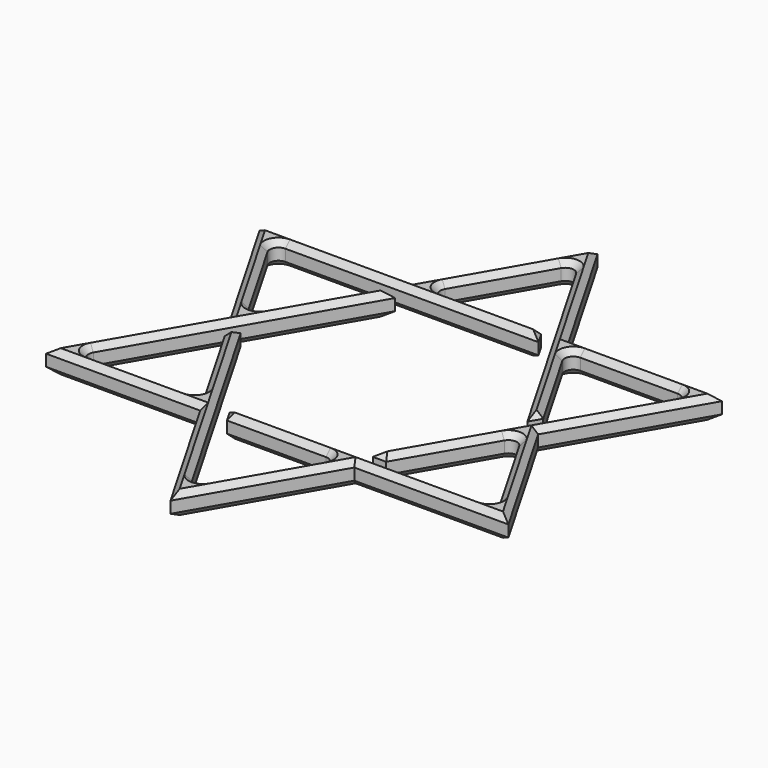
from build123d import *

# Parameters (mm, degrees)
F1_DEPTH = 12.7
F2_SIZE  = 3.17499
F3_SIZE  = 3.17499


# Not quite as in the source:
# - a fillet or chamfer is up to 0.001 mm smaller than in the source, because OpenCascade refuses the exact size


with BuildPart() as f1:
    # F0 (on Top) → F1 (new body)
    with BuildSketch(Plane.XY):
        Polygon((42.3333333333, 73.3234841871), (0, 146.6469683742), (-42.3333333333, 73.3234841871), (-127, 73.3234841871), (-84.6666666667, 0), (-127, -73.3234841871), (-42.3333333333, -73.3234841871), (0, -146.6469683742), (42.3333333333, -73.3234841871), (127, -73.3234841871), (84.6666666667, 0), (127, 73.3234841871), align=None)
        with BuildLine():
            ThreePointArc((107.7525859006, 66.9734850526), (111.8770318861, 64.5922350526), (111.8770318861, 59.8297350526))
            Line((111.8770318861, 59.8297350526), (42.3333325205, -60.623485595))
            Line((42.3333325205, -60.623485595), (49.6656809392, -60.623485595))
            Line((49.6656809392, -60.623485595), (76.8760464718, -13.49375))
            ThreePointArc((76.8760464718, -13.49375), (81.0004924573, -11.1125), (85.1249384428, -13.49375))
            Line((85.1249384428, -13.49375), (111.8770318861, -59.8297350526))
            ThreePointArc((111.8770318861, -59.8297350526), (111.8770318861, -64.5922350526), (107.7525859006, -66.9734850526))
            Line((107.7525859006, -66.9734850526), (-31.3348102056, -66.9734850526))
            Line((-31.3348102056, -66.9734850526), (-27.6686364959, -73.3234841871))
            Line((-27.6686364959, -73.3234841871), (26.7520929436, -73.3234841871))
            ThreePointArc((26.7520929436, -73.3234841871), (30.8765389291, -75.7047341871), (30.8765389291, -80.4672341871))
            Line((30.8765389291, -80.4672341871), (4.1244459855, -126.8032183742))
            ThreePointArc((4.1244459855, -126.8032183742), (0, -129.1844683742), (-4.1244459855, -126.8032183742))
            Line((-4.1244459855, -126.8032183742), (-73.6681446525, -6.3499989368))
            Line((-73.6681446525, -6.3499989368), (-77.3343188618, -12.6999989368))
            Line((-77.3343188618, -12.6999989368), (-50.1239530285, -59.8297350526))
            ThreePointArc((-50.1239530285, -59.8297350526), (-50.1239530285, -64.5922350526), (-54.2483990141, -66.9734850526))
            Line((-54.2483990141, -66.9734850526), (-107.7525871283, -66.9734850526))
            ThreePointArc((-107.7525871283, -66.9734850526), (-111.8770331138, -64.5922350526), (-111.8770331138, -59.8297350526))
            Line((-111.8770331138, -59.8297350526), (-42.3333337482, 60.623485595))
            Line((-42.3333337482, 60.623485595), (-49.6656809392, 60.623485595))
            Line((-49.6656809392, 60.623485595), (-76.8760464718, 13.49375))
            ThreePointArc((-76.8760464718, 13.49375), (-81.0004924573, 11.1125), (-85.1249384428, 13.49375))
            Line((-85.1249384428, 13.49375), (-111.8770318861, 59.8297350526))
            ThreePointArc((-111.8770318861, 59.8297350526), (-111.8770318861, 64.5922350526), (-107.7525859006, 66.9734850526))
            Line((-107.7525859006, 66.9734850526), (31.3348102056, 66.9734850526))
            Line((31.3348102056, 66.9734850526), (27.6686364959, 73.3234841871))
            Line((27.6686364959, 73.3234841871), (-26.7520941713, 73.3234841871))
            ThreePointArc((-26.7520941713, 73.3234841871), (-30.8765401568, 75.7047341871), (-30.8765401568, 80.4672341871))
            Line((-30.8765401568, 80.4672341871), (-4.1244465994, 126.8032194374))
            ThreePointArc((-4.1244465994, 126.8032194374), (-6.138e-07, 129.1844694374), (4.1244453717, 126.8032194374))
            Line((4.1244453717, 126.8032194374), (73.6681440386, 6.35))
            Line((73.6681440386, 6.35), (77.334318248, 12.7))
            Line((77.334318248, 12.7), (50.1239530285, 59.8297350526))
            ThreePointArc((50.1239530285, 59.8297350526), (50.1239530285, 64.5922350526), (54.248399014, 66.9734850526))
            Line((54.248399014, 66.9734850526), (107.7525859006, 66.9734850526))
        make_face(mode=Mode.SUBTRACT)
    extrude(amount=F1_DEPTH)

    # F2 (size 3.175 in the source; OpenCascade refuses exactly that, so slightly less here)
    f2_edges = [f1.edges().sort_by_distance(p)[0] for p in [
        (105.833333, -36.661742, 12.7),
        (105.833333, 36.661742, 12.7),
        (84.666667, 73.323484, 12.7),
        (21.166667, 109.985226, 12.7),
        (-21.166667, 109.985226, 12.7),
        (-84.666667, 73.323484, 12.7),
        (-105.833333, 36.661742, 12.7),
        (-105.833333, -36.661742, 12.7),
        (-84.666667, -73.323484, 12.7),
        (-21.166667, -109.985226, 12.7),
        (21.166667, -109.985226, 12.7),
        (84.666667, -73.323484, 12.7),
        (38.896295, 66.57661, 12.7),
        (75.501231, 9.525, 12.7),
        (63.729136, 36.264868, 12.7),
        (50.123953, 64.592235, 12.7),
        (81.000492, 66.973485, 12.7),
        (111.877032, 64.592235, 12.7),
        (77.105182, -0.396875, 12.7),
        (45.999507, -60.623486, 12.7),
        (63.270864, -37.058618, 12.7),
        (81.000492, -11.1125, 12.7),
        (98.500985, -36.661743, 12.7),
        (111.877032, -64.592235, 12.7),
        (38.208888, -66.973485, 12.7),
        (-29.501723, -70.148485, 12.7),
        (-0.458272, -73.323484, 12.7),
        (30.876539, -75.704734, 12.7),
        (17.500492, -103.635226, 12.7),
        (0, -129.184468, 12.7),
        (-38.896295, -66.576609, 12.7),
        (-75.501232, -9.524999, 12.7),
        (-63.729136, -36.264867, 12.7),
        (-50.123953, -64.592235, 12.7),
        (-81.000493, -66.973485, 12.7),
        (-111.877033, -64.592235, 12.7),
        (-77.105183, 0.396875, 12.7),
        (-45.999507, 60.623486, 12.7),
        (-63.270864, 37.058618, 12.7),
        (-81.000492, 11.1125, 12.7),
        (-98.500985, 36.661743, 12.7),
        (-111.877032, 64.592235, 12.7),
        (-38.208888, 66.973485, 12.7),
        (29.501723, 70.148485, 12.7),
        (0.458271, 73.323484, 12.7),
        (-30.87654, 75.704734, 12.7),
        (-17.500493, 103.635227, 12.7),
        (-1e-06, 129.184469, 12.7),
    ]]
    chamfer(f2_edges, length=F2_SIZE)

    # F3 (size 3.175 in the source; OpenCascade refuses exactly that, so slightly less here)
    f3_edges = [f1.edges().sort_by_distance(p)[0] for p in [
        (105.833333, -36.661742, 0),
        (105.833333, 36.661742, 0),
        (84.666667, 73.323484, 0),
        (21.166667, 109.985226, 0),
        (-21.166667, 109.985226, 0),
        (-84.666667, 73.323484, 0),
        (-105.833333, 36.661742, 0),
        (-105.833333, -36.661742, 0),
        (-84.666667, -73.323484, 0),
        (-21.166667, -109.985226, 0),
        (21.166667, -109.985226, 0),
        (84.666667, -73.323484, 0),
        (38.896295, 66.57661, 0),
        (75.501231, 9.525, 0),
        (63.729136, 36.264868, 0),
        (50.123953, 64.592235, 0),
        (81.000492, 66.973485, 0),
        (111.877032, 64.592235, 0),
        (77.105182, -0.396875, 0),
        (45.999507, -60.623486, 0),
        (63.270864, -37.058618, 0),
        (81.000492, -11.1125, 0),
        (98.500985, -36.661743, 0),
        (111.877032, -64.592235, 0),
        (38.208888, -66.973485, 0),
        (-29.501723, -70.148485, 0),
        (-0.458272, -73.323484, 0),
        (30.876539, -75.704734, 0),
        (17.500492, -103.635226, 0),
        (0, -129.184468, 0),
        (-38.896295, -66.576609, 0),
        (-75.501232, -9.524999, 0),
        (-63.729136, -36.264867, 0),
        (-50.123953, -64.592235, 0),
        (-81.000493, -66.973485, 0),
        (-111.877033, -64.592235, 0),
        (-77.105183, 0.396875, 0),
        (-45.999507, 60.623486, 0),
        (-63.270864, 37.058618, 0),
        (-81.000492, 11.1125, 0),
        (-98.500985, 36.661743, 0),
        (-111.877032, 64.592235, 0),
        (-38.208888, 66.973485, 0),
        (29.501723, 70.148485, 0),
        (0.458271, 73.323484, 0),
        (-30.87654, 75.704734, 0),
        (-17.500493, 103.635227, 0),
        (-1e-06, 129.184469, 0),
    ]]
    chamfer(f3_edges, length=F3_SIZE)


solid = f1.part
